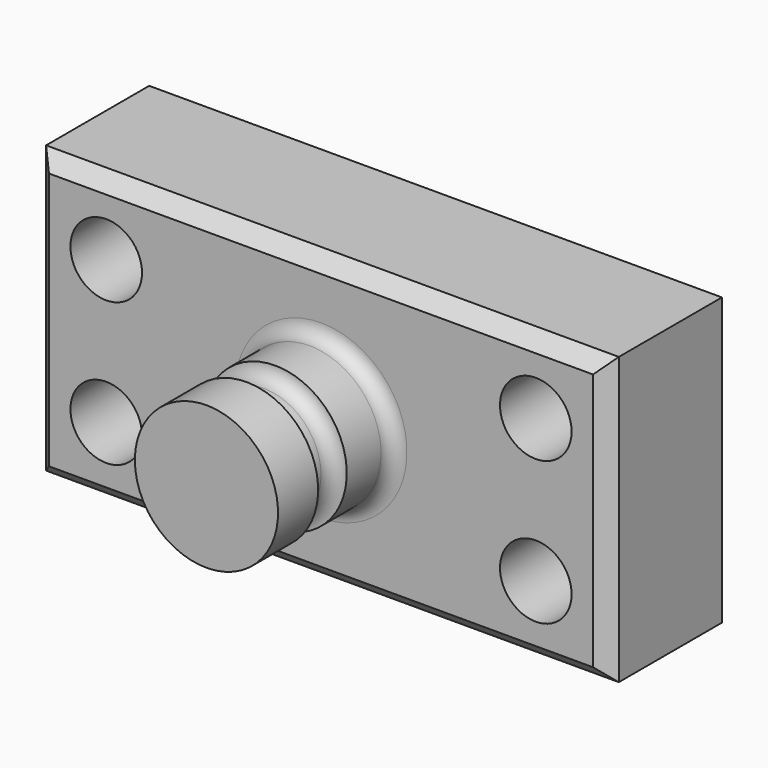
from build123d import *

# Parameters (mm, degrees)
F0_W     = 101.6
F0_H     = 50.8
F1_DEPTH = 25.4
F2_R     = 6.35
F3_DEPTH = 25.401
F4_W     = 12.7
F4_H     = 25.4
F6_W     = 10.16
F6_H     = 6.35
F8_R     = 2.53999
F9_SIZE  = 2.54


# Not quite as in the source:
# - a fillet or chamfer is up to 0.001 mm smaller than in the source, because OpenCascade refuses the exact size


with BuildPart() as f1:
    # F0 (on Front) → F1 (new body)
    with BuildSketch(Plane.XZ):
        Rectangle(F0_W, F0_H)
    extrude(amount=F1_DEPTH)

    # F2 (on face) → F3 (cut, through all)
    with BuildSketch(Plane.XZ.offset(25.4)):
        with Locations((-38.1, 12.7)):
            Circle(F2_R)
        with Locations((-38.1, -12.7)):
            Circle(F2_R)
        with Locations((38.1, 12.7)):
            Circle(F2_R)
        with Locations((38.1, -12.7)):
            Circle(F2_R)
    extrude(amount=-F3_DEPTH, mode=Mode.SUBTRACT)

    # F4 (on Top) → F5 (revolve)
    with BuildSketch(Plane.XY):
        with Locations((-6.35, -38.1)):
            Rectangle(F4_W, F4_H)
    revolve(axis=Axis((0, -38.1, 0), (0, -1, 0)))

    # F6 (on Top) → F7 (revolve, cut)
    with BuildSketch(Plane.XY):
        with Locations((-15.24, -38.735)):
            Rectangle(F6_W, F6_H)
    revolve(axis=Axis((0, -57.4092715979, 0), (0, -1, 0)), mode=Mode.SUBTRACT)

    # F8 (radius 2.54 in the source; OpenCascade refuses exactly that, so slightly less here)
    f8_edges = [f1.edges().sort_by_distance(p)[0] for p in [
        (12.7, -25.4, 0),
        (10.16, -35.56, 0),
        (10.16, -41.91, 0),
        (-10.16, -38.735, 0),
    ]]
    fillet(f8_edges, radius=F8_R)

    # F9
    f9_edges = [f1.edges().sort_by_distance(p)[0] for p in [
        (-50.8, -25.4, 0),
        (0, -25.4, 25.4),
        (50.8, -25.4, 0),
        (0, -25.4, -25.4),
    ]]
    chamfer(f9_edges, length=F9_SIZE)


solid = f1.part
